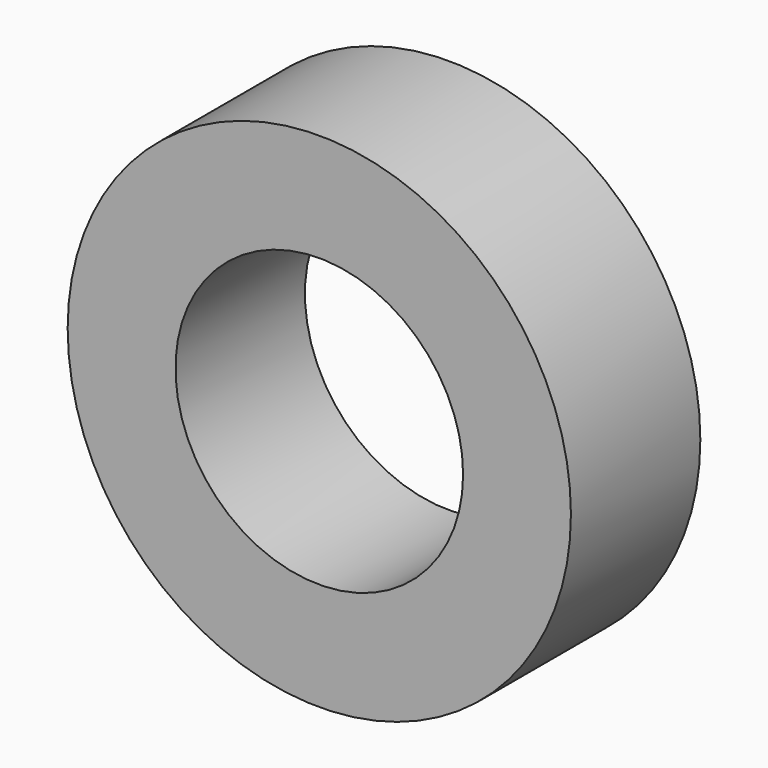
from build123d import *

# Parameters (mm, degrees)
F0_R        = 44.45
F0_R_2      = 25.4
F2_DEPTH    = 3.175
F2_FACE_R   = 44.45
F2_FACE_R_2 = 25.4
F3_DEPTH    = 25.4


# Not quite as in the source:
# - the program builds the solid bodies; features that only make, move or delete a surface that nothing else refers to are left out


with BuildPart() as f2:
    # F0 (on Front) → F2 (new body)
    with BuildSketch(Plane.XZ):
        Circle(F0_R)
        Circle(F0_R_2, mode=Mode.SUBTRACT)
    extrude(amount=F2_DEPTH)

    # F0 (on Front) + F2_face (on face) → F3 (join)
    with BuildSketch(Plane.XZ):
        Circle(F0_R)
        Circle(F0_R_2, mode=Mode.SUBTRACT)
    with BuildSketch(Plane.XZ.offset(3.175)):
        Circle(F2_FACE_R)
        Circle(F2_FACE_R_2, mode=Mode.SUBTRACT)
    extrude(amount=F3_DEPTH)


solid = f2.part
